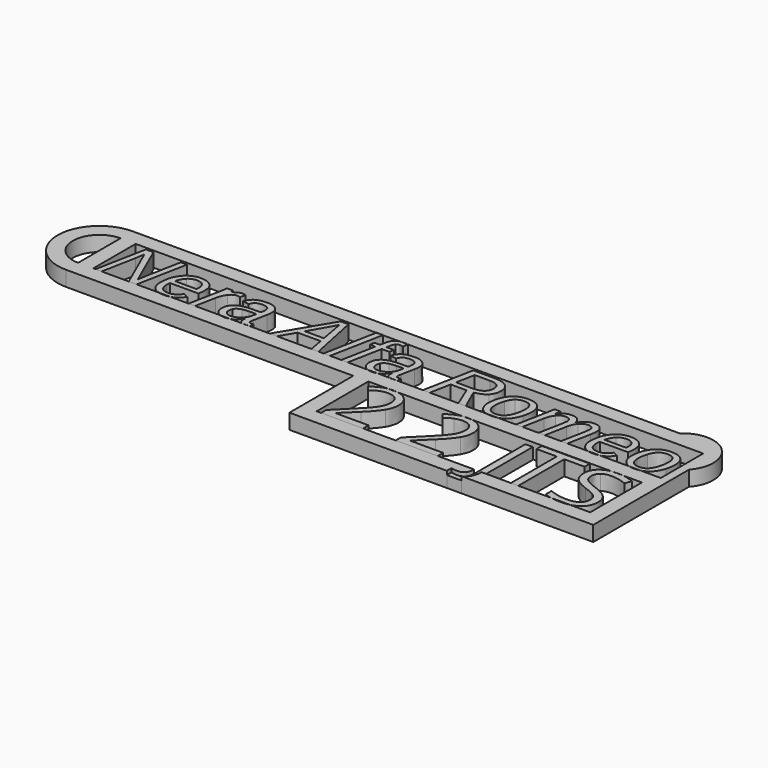
from build123d import *

# Parameters (mm, degrees)
F1_DEPTH = 2
F2_DEPTH = 2
F3_DEPTH = 0.5


with BuildPart() as f1:
    # F0 (on Top) → F1 (new body)
    with BuildSketch(Plane.XY):
        with BuildLine():
            Line((-9.0088317637, 8.9224354902), (-10.3058150991, 2.2276903254))
            Line((-10.3058150991, 2.2276903254), (-9.4984315691, 2.2276903254))
            Line((-9.4984315691, 2.2276903254), (-8.637830669, 6.7085928919))
            add(Edge.make_bspline(
                [(-8.438645655, 7.9766867978), (-8.543559899, 7.1647417789), (-8.637830669, 6.7085928919)],
                knots=[0, 0, 0, 1, 1, 1], degree=2))
            Line((-8.438645655, 7.9766867978), (-5.9161423099, 2.2276903254))
            Line((-5.9161423099, 2.2276903254), (-4.8700408624, 2.2276903254))
            Line((-4.8700408624, 2.2276903254), (-3.573057527, 8.9224354902))
            Line((-3.573057527, 8.9224354902), (-4.3895640347, 8.9224354902))
            Line((-4.3895640347, 8.9224354902), (-5.2501649349, 4.4993117826))
            add(Edge.make_bspline(
                [(-5.4645549118, 3.1491110771), (-5.339874216, 4.0477243845), (-5.2501649349, 4.4993117826)],
                knots=[0, 0, 0, 1, 1, 1], degree=2))
            Line((-5.4645549118, 3.1491110771), (-8.0007427235, 8.9224354902))
            Line((-8.0007427235, 8.9224354902), (-9.0088317637, 8.9224354902))
        make_face()
        with BuildLine():
            add(Edge.make_bspline(
                [(-1.9696861122, 2.2276903254), (-2.4147037445, 2.3571969005), (-2.7192988602, 2.6617920161)],
                knots=[0.4251761387, 0.4251761387, 0.4251761387, 1, 1, 1], degree=2))
            Line((-1.9696861122, 2.2276903254), (-0.4300085657, 2.2276903254))
            add(Edge.make_bspline(
                [(0.0601683579, 2.4177523616), (-0.1648991002, 2.2973748876), (-0.4300085657, 2.2276903254)],
                knots=[0, 0, 0, 0.4211162613, 0.4211162613, 0.4211162613], degree=2))
            add(Edge.make_bspline(
                [(0.941295958, 3.3254886467), (0.5946228038, 2.7036056641), (0.0601683579, 2.4177523616)],
                knots=[0, 0, 0, 1, 1, 1], degree=2))
            Line((0.941295958, 3.3254886467), (0.285962057, 3.6250264159))
            add(Edge.make_bspline(
                [(-0.2994290147, 3.001622937), (0.076133569, 3.2296973805), (0.285962057, 3.6250264159)],
                knots=[0, 0, 0, 1, 1, 1], degree=2))
            add(Edge.make_bspline(
                [(-1.1357019742, 2.7735484935), (-0.6749915983, 2.7735484935), (-0.2994290147, 3.001622937)],
                knots=[0, 0, 0, 1, 1, 1], degree=2))
            add(Edge.make_bspline(
                [(-2.0875326517, 3.1110986698), (-1.7712694234, 2.7735484935), (-1.1357019742, 2.7735484935)],
                knots=[0, 0, 0, 1, 1, 1], degree=2))
            add(Edge.make_bspline(
                [(-2.40379588, 4.0811753028), (-2.40379588, 3.4486488462), (-2.0875326517, 3.1110986698)],
                knots=[0, 0, 0, 1, 1, 1], degree=2))
            add(Edge.make_bspline(
                [(-2.3612219839, 4.6179104932), (-2.3901114134, 4.4521763976), (-2.40379588, 4.0811753028)],
                knots=[0, 0, 0, 1, 1, 1], degree=2))
            Line((-2.3612219839, 4.6179104932), (1.3594324377, 4.6179104932))
            add(Edge.make_bspline(
                [(1.4734696595, 5.5925486151), (1.4734696595, 5.0923053357), (1.3594324377, 4.6179104932)],
                knots=[0, 0, 0, 1, 1, 1], degree=2))
            add(Edge.make_bspline(
                [(0.9314127321, 6.9746797427), (1.4734696595, 6.4850799373), (1.4734696595, 5.5925486151)],
                knots=[0, 0, 0, 1, 1, 1], degree=2))
            add(Edge.make_bspline(
                [(-0.5837618209, 7.4642795481), (0.3893558047, 7.4642795481), (0.9314127321, 6.9746797427)],
                knots=[0, 0, 0, 1, 1, 1], degree=2))
            add(Edge.make_bspline(
                [(-1.9620917078, 7.0438623239), (-1.3485714548, 7.4642795481), (-0.5837618209, 7.4642795481)],
                knots=[0, 0, 0, 1, 1, 1], degree=2))
            add(Edge.make_bspline(
                [(-2.912401889, 5.8654776992), (-2.5756119608, 6.6234450997), (-1.9620917078, 7.0438623239)],
                knots=[0, 0, 0, 1, 1, 1], degree=2))
            add(Edge.make_bspline(
                [(-3.2491918173, 4.1526386285), (-3.2491918173, 5.1075102986), (-2.912401889, 5.8654776992)],
                knots=[0, 0, 0, 1, 1, 1], degree=2))
            add(Edge.make_bspline(
                [(-2.7192988602, 2.6617920161), (-3.2491918173, 3.1916849732), (-3.2491918173, 4.1526386285)],
                knots=[0, 0, 0, 1, 1, 1], degree=2))
        make_face()
        with BuildLine():
            Line((0.6235122334, 5.6153560594), (0.6037457816, 5.2732443942))
            Line((0.6037457816, 5.2732443942), (-2.2471847621, 5.2732443942))
            add(Edge.make_bspline(
                [(-1.6359452536, 6.425780582), (-2.0708071925, 6.0198080726), (-2.2471847621, 5.2732443942)],
                knots=[0, 0, 0, 1, 1, 1], degree=2))
            add(Edge.make_bspline(
                [(-0.5655158654, 6.8317530914), (-1.2010833146, 6.8317530914), (-1.6359452536, 6.425780582)],
                knots=[0, 0, 0, 1, 1, 1], degree=2))
            add(Edge.make_bspline(
                [(0.3163719828, 6.5185308557), (0.0092317322, 6.8317530914), (-0.5655158654, 6.8317530914)],
                knots=[0, 0, 0, 1, 1, 1], degree=2))
            add(Edge.make_bspline(
                [(0.6235122334, 5.6153560594), (0.6235122334, 6.20530862), (0.3163719828, 6.5185308557)],
                knots=[0, 0, 0, 1, 1, 1], degree=2))
        make_face(mode=Mode.SUBTRACT)
        with BuildLine():
            Line((2.7658915059, 6.1718577016), (1.9949998869, 2.2276903254))
            Line((1.9949998869, 2.2276903254), (2.8510392982, 2.2276903254))
            Line((2.8510392982, 2.2276903254), (3.3740900219, 4.9083252846))
            add(Edge.make_bspline(
                [(3.9169071975, 6.2235545754), (3.5154961769, 5.7005038517), (3.3740900219, 4.9083252846)],
                knots=[0, 0, 0, 1, 1, 1], degree=2))
            add(Edge.make_bspline(
                [(4.8185614974, 6.7466052992), (4.318318218, 6.7466052992), (3.9169071975, 6.2235545754)],
                knots=[0, 0, 0, 1, 1, 1], degree=2))
            add(Edge.make_bspline(
                [(5.2458209549, 6.6842649513), (5.0359924669, 6.7466052992), (4.8185614974, 6.7466052992)],
                knots=[0, 0, 0, 1, 1, 1], degree=2))
            Line((5.2458209549, 6.6842649513), (5.4024320728, 7.3973777113))
            add(Edge.make_bspline(
                [(4.9508446747, 7.4642795481), (5.1697961404, 7.4642795481), (5.4024320728, 7.3973777113)],
                knots=[0, 0, 0, 1, 1, 1], degree=2))
            add(Edge.make_bspline(
                [(4.2483753887, 7.2073156751), (4.5524746467, 7.4642795481), (4.9508446747, 7.4642795481)],
                knots=[0, 0, 0, 1, 1, 1], degree=2))
            add(Edge.make_bspline(
                [(4.1290557119, 7.0925359614), (4.1889189826, 7.1570750119), (4.2483753887, 7.2073156751)],
                knots=[0.8044835543, 0.8044835543, 0.8044835543, 1, 1, 1], degree=2))
            add(Edge.make_bspline(
                [(3.6295333987, 6.3193458417), (3.8827387504, 6.8269797595), (4.1290557119, 7.0925359614)],
                knots=[0, 0, 0, 0.8044835543, 0.8044835543, 0.8044835543], degree=2))
            Line((3.6295333987, 6.3193458417), (3.6112874432, 6.3193458417))
            Line((3.6112874432, 6.3193458417), (3.7334290708, 7.0925359614))
            Line((3.7334290708, 7.0925359614), (3.7770215388, 7.3684882818))
            Line((3.7770215388, 7.3684882818), (2.9696380088, 7.3684882818))
            Line((2.9696380088, 7.3684882818), (2.8844902166, 6.8271916026))
            Line((2.8844902166, 6.8271916026), (2.7658915059, 6.1718577016))
        make_face()
        with BuildLine():
            Line((9.0913622365, 2.2276903254), (9.9547242293, 2.2276903254))
            add(Edge.make_bspline(
                [(10.0870811422, 2.2565797549), (10.0204903416, 2.2404169392), (9.9547242293, 2.2276903254)],
                knots=[0, 0, 0, 0.2125992126, 0.2125992126, 0.2125992126], degree=2))
            Line((10.0870811422, 2.2565797549), (10.153982979, 2.7887534564))
            add(Edge.make_bspline(
                [(9.8681296765, 2.755302538), (9.9973718611, 2.755302538), (10.153982979, 2.7887534564)],
                knots=[0, 0, 0, 1, 1, 1], degree=2))
            add(Edge.make_bspline(
                [(9.4834441151, 3.1019756921), (9.4834441151, 2.755302538), (9.8681296765, 2.755302538)],
                knots=[0, 0, 0, 1, 1, 1], degree=2))
            add(Edge.make_bspline(
                [(9.535140989, 3.5201121718), (9.4834441151, 3.2920377283), (9.4834441151, 3.1019756921)],
                knots=[0, 0, 0, 1, 1, 1], degree=2))
            Line((9.535140989, 3.5201121718), (9.8878961283, 5.3158182903))
            add(Edge.make_bspline(
                [(9.9776054094, 6.0623819687), (9.9776054094, 5.7582827107), (9.8878961283, 5.3158182903)],
                knots=[0, 0, 0, 1, 1, 1], degree=2))
            add(Edge.make_bspline(
                [(9.5047310632, 7.0841554756), (9.9776054094, 6.7040314031), (9.9776054094, 6.0623819687)],
                knots=[0, 0, 0, 1, 1, 1], degree=2))
            add(Edge.make_bspline(
                [(8.2199116981, 7.4642795481), (9.031856717, 7.4642795481), (9.5047310632, 7.0841554756)],
                knots=[0, 0, 0, 1, 1, 1], degree=2))
            add(Edge.make_bspline(
                [(6.7959669226, 7.1480163198), (7.3258598796, 7.4642795481), (8.2199116981, 7.4642795481)],
                knots=[0, 0, 0, 1, 1, 1], degree=2))
            add(Edge.make_bspline(
                [(6.0532044849, 6.1338452943), (6.2660739655, 6.8317530914), (6.7959669226, 7.1480163198)],
                knots=[0, 0, 0, 1, 1, 1], degree=2))
            Line((6.0532044849, 6.1338452943), (6.8986004221, 5.9954801319))
            add(Edge.make_bspline(
                [(7.3167369019, 6.6112811294), (7.0263221105, 6.4090551228), (6.8986004221, 5.9954801319)],
                knots=[0, 0, 0, 1, 1, 1], degree=2))
            add(Edge.make_bspline(
                [(8.1727763131, 6.813507136), (7.6071516933, 6.813507136), (7.3167369019, 6.6112811294)],
                knots=[0, 0, 0, 1, 1, 1], degree=2))
            add(Edge.make_bspline(
                [(8.8706841103, 6.6067196405), (8.6182817261, 6.813507136), (8.1727763131, 6.813507136)],
                knots=[0, 0, 0, 1, 1, 1], degree=2))
            add(Edge.make_bspline(
                [(9.1230864944, 5.9665907024), (9.1230864944, 6.3999321451), (8.8706841103, 6.6067196405)],
                knots=[0, 0, 0, 1, 1, 1], degree=2))
            add(Edge.make_bspline(
                [(9.031856717, 5.3644741716), (9.1230864944, 5.8297460363), (9.1230864944, 5.9665907024)],
                knots=[0, 0, 0, 1, 1, 1], degree=2))
            Line((9.031856717, 5.3644741716), (7.9294969067, 5.3492692087))
            add(Edge.make_bspline(
                [(5.922441804, 4.8794358551), (6.551927268, 5.3310232532), (7.9294969067, 5.3492692087)],
                knots=[0, 0, 0, 1, 1, 1], degree=2))
            add(Edge.make_bspline(
                [(5.2929563399, 3.5490016014), (5.2929563399, 4.427848457), (5.922441804, 4.8794358551)],
                knots=[0, 0, 0, 1, 1, 1], degree=2))
            add(Edge.make_bspline(
                [(5.7088120752, 2.5317895833), (5.2929563399, 2.9316801076), (5.2929563399, 3.5490016014)],
                knots=[0, 0, 0, 1, 1, 1], degree=2))
            add(Edge.make_bspline(
                [(6.1982625562, 2.2276903254), (5.9211346878, 2.327618296), (5.7088120752, 2.5317895833)],
                knots=[0.4894320446, 0.4894320446, 0.4894320446, 1, 1, 1], degree=2))
            Line((6.1982625562, 2.2276903254), (7.4753742359, 2.2276903254))
            add(Edge.make_bspline(
                [(7.8108981961, 2.3721374729), (7.6551145583, 2.2835985708), (7.4753742359, 2.2276903254)],
                knots=[0, 0, 0, 0.3685459817, 0.3685459817, 0.3685459817], degree=2))
            add(Edge.make_bspline(
                [(8.6289252001, 3.211451425), (8.2335961647, 2.6123758867), (7.8108981961, 2.3721374729)],
                knots=[0, 0, 0, 1, 1, 1], degree=2))
            Line((8.6289252001, 3.211451425), (8.6562941334, 3.211451425))
            Line((8.6562941334, 3.211451425), (8.633486689, 2.907352167))
            add(Edge.make_bspline(
                [(8.8349524474, 2.3630144952), (8.633486689, 2.54547405), (8.633486689, 2.907352167)],
                knots=[0, 0, 0, 1, 1, 1], degree=2))
            add(Edge.make_bspline(
                [(9.0913622365, 2.2276903254), (8.9340202076, 2.2732927501), (8.8349524474, 2.3630144952)],
                knots=[0.5082650227, 0.5082650227, 0.5082650227, 1, 1, 1], degree=2))
        make_face()
        with BuildLine():
            Line((7.9720708029, 4.7562756556), (8.9178194952, 4.7745216111))
            Line((8.9178194952, 4.7745216111), (8.7900978069, 4.1800075617))
            add(Edge.make_bspline(
                [(8.4715538341, 3.4965444793), (8.7140729924, 3.8150884521), (8.7900978069, 4.1800075617)],
                knots=[0, 0, 0, 1, 1, 1], degree=2))
            add(Edge.make_bspline(
                [(7.8587938293, 2.981096237), (8.2290346759, 3.1780005066), (8.4715538341, 3.4965444793)],
                knots=[0, 0, 0, 1, 1, 1], degree=2))
            add(Edge.make_bspline(
                [(7.0263221105, 2.7841919675), (7.4885529827, 2.7841919675), (7.8587938293, 2.981096237)],
                knots=[0, 0, 0, 1, 1, 1], degree=2))
            add(Edge.make_bspline(
                [(6.431047813, 3.006944674), (6.6614030009, 2.7841919675), (7.0263221105, 2.7841919675)],
                knots=[0, 0, 0, 1, 1, 1], degree=2))
            add(Edge.make_bspline(
                [(6.200692625, 3.5870140086), (6.200692625, 3.2296973805), (6.431047813, 3.006944674)],
                knots=[0, 0, 0, 1, 1, 1], degree=2))
            add(Edge.make_bspline(
                [(6.3025658765, 4.0880175362), (6.200692625, 3.8819902889), (6.200692625, 3.5870140086)],
                knots=[0, 0, 0, 1, 1, 1], degree=2))
            add(Edge.make_bspline(
                [(6.5823371938, 4.4301292014), (6.4044391279, 4.2940447834), (6.3025658765, 4.0880175362)],
                knots=[0, 0, 0, 1, 1, 1], degree=2))
            add(Edge.make_bspline(
                [(7.0833407214, 4.653642156), (6.7602352597, 4.5662136194), (6.5823371938, 4.4301292014)],
                knots=[0, 0, 0, 1, 1, 1], degree=2))
            add(Edge.make_bspline(
                [(7.9720708029, 4.7562756556), (7.406446183, 4.7410706927), (7.0833407214, 4.653642156)],
                knots=[0, 0, 0, 1, 1, 1], degree=2))
        make_face(mode=Mode.SUBTRACT)
        Polygon((18.2308592714, 2.2276903254), (19.156841512, 2.2276903254), (17.7701488956, 8.9224354902), (16.7377319147, 8.9224354902), (12.7084167462, 2.2276903254), (13.6967393347, 2.2276903254), (14.8371115522, 4.1860895469), (17.8735426433, 4.1860895469), align=None)
        with BuildLine():
            add(Edge.make_bspline(
                [(17.1330609501, 8.2382121597), (17.0707206022, 8.1150519602), (16.9566833804, 7.9105452092)],
                knots=[0, 0, 0, 1, 1, 1], degree=2))
            Line((17.1330609501, 8.2382121597), (17.2562211495, 7.5205379108))
            Line((17.2562211495, 7.5205379108), (17.741259466, 4.8931203217))
            Line((17.741259466, 4.8931203217), (15.2370020764, 4.8931203217))
            add(Edge.make_bspline(
                [(16.9566833804, 7.9105452092), (16.8426461587, 7.7060384582), (15.2370020764, 4.8931203217)],
                knots=[0, 0, 0, 1, 1, 1], degree=2))
        make_face(mode=Mode.SUBTRACT)
        Polygon((22.05210839, 9.2341372296), (21.1960984838, 9.2341372296), (19.8365033537, 2.2276903254), (20.687981276, 2.2276903254), align=None)
        with BuildLine():
            Line((25.3320137021, 9.2341372296), (24.3199696419, 9.2341372296))
            add(Edge.make_bspline(
                [(24.0421960918, 9.1436677004), (24.1663926885, 9.2009645839), (24.3199696419, 9.2341372296)],
                knots=[0, 0, 0, 0.4210392667, 0.4210392667, 0.4210392667], degree=2))
            add(Edge.make_bspline(
                [(23.5693217456, 8.7445374242), (23.7472198115, 9.0075832824), (24.0421960918, 9.1436677004)],
                knots=[0, 0, 0, 1, 1, 1], degree=2))
            add(Edge.make_bspline(
                [(23.2819479468, 7.9493178646), (23.3914236796, 8.4814915661), (23.5693217456, 8.7445374242)],
                knots=[0, 0, 0, 1, 1, 1], degree=2))
            Line((23.2819479468, 7.9493178646), (23.1724722139, 7.3684882818))
            Line((23.1724722139, 7.3684882818), (22.4502364761, 7.3684882818))
            Line((22.4502364761, 7.3684882818), (22.3270762767, 6.7466052992))
            Line((22.3270762767, 6.7466052992), (23.0493120144, 6.7466052992))
            Line((23.0493120144, 6.7466052992), (22.1704651588, 2.2276903254))
            Line((22.1704651588, 2.2276903254), (23.0249840738, 2.2276903254))
            Line((23.0249840738, 2.2276903254), (23.9038309294, 6.7466052992))
            Line((23.9038309294, 6.7466052992), (24.9073584808, 6.7466052992))
            Line((24.9073584808, 6.7466052992), (25.0305186803, 7.3684882818))
            Line((25.0305186803, 7.3684882818), (24.0285116252, 7.3684882818))
            Line((24.0285116252, 7.3684882818), (24.1182209063, 7.8291986577))
            add(Edge.make_bspline(
                [(24.3721437867, 8.454882881), (24.2124916762, 8.3005525076), (24.1182209063, 7.8291986577)],
                knots=[0, 0, 0, 1, 1, 1], degree=2))
            add(Edge.make_bspline(
                [(24.8313336663, 8.6092132544), (24.5317958971, 8.6092132544), (24.3721437867, 8.454882881)],
                knots=[0, 0, 0, 1, 1, 1], degree=2))
            Line((24.8313336663, 8.6092132544), (25.0487646357, 8.6000902767))
            Line((25.0487646357, 8.6000902767), (25.2631546126, 8.5712008472))
            Line((25.2631546126, 8.5712008472), (25.3863148121, 9.2219732593))
            add(Edge.make_bspline(
                [(25.3320137021, 9.2341372296), (25.3598728303, 9.2284142549), (25.3863148121, 9.2219732593)],
                knots=[0.8885233166, 0.8885233166, 0.8885233166, 1, 1, 1], degree=2))
        make_face()
        with BuildLine():
            add(Edge.make_bspline(
                [(25.6697380458, 2.2276903254), (25.3926101774, 2.327618296), (25.1802875648, 2.5317895833)],
                knots=[0.4894320446, 0.4894320446, 0.4894320446, 1, 1, 1], degree=2))
            Line((25.6697380458, 2.2276903254), (26.9468497255, 2.2276903254))
            add(Edge.make_bspline(
                [(27.2823736857, 2.3721374729), (27.1265900479, 2.2835985708), (26.9468497255, 2.2276903254)],
                knots=[0, 0, 0, 0.3685459817, 0.3685459817, 0.3685459817], degree=2))
            add(Edge.make_bspline(
                [(28.1004006897, 3.211451425), (27.7050716543, 2.6123758867), (27.2823736857, 2.3721374729)],
                knots=[0, 0, 0, 1, 1, 1], degree=2))
            Line((28.1004006897, 3.211451425), (28.127769623, 3.211451425))
            Line((28.127769623, 3.211451425), (28.1049621786, 2.907352167))
            add(Edge.make_bspline(
                [(28.306427937, 2.3630144952), (28.1049621786, 2.54547405), (28.1049621786, 2.907352167)],
                knots=[0, 0, 0, 1, 1, 1], degree=2))
            add(Edge.make_bspline(
                [(28.5628377261, 2.2276903254), (28.4054956972, 2.2732927501), (28.306427937, 2.3630144952)],
                knots=[0.5082650227, 0.5082650227, 0.5082650227, 1, 1, 1], degree=2))
            Line((28.5628377261, 2.2276903254), (29.4261997189, 2.2276903254))
            add(Edge.make_bspline(
                [(29.5585566318, 2.2565797549), (29.4919658312, 2.2404169392), (29.4261997189, 2.2276903254)],
                knots=[0, 0, 0, 0.2125992126, 0.2125992126, 0.2125992126], degree=2))
            Line((29.5585566318, 2.2565797549), (29.6254584686, 2.7887534564))
            add(Edge.make_bspline(
                [(29.3396051661, 2.755302538), (29.4688473507, 2.755302538), (29.6254584686, 2.7887534564)],
                knots=[0, 0, 0, 1, 1, 1], degree=2))
            add(Edge.make_bspline(
                [(28.9549196047, 3.1019756921), (28.9549196047, 2.755302538), (29.3396051661, 2.755302538)],
                knots=[0, 0, 0, 1, 1, 1], degree=2))
            add(Edge.make_bspline(
                [(29.0066164786, 3.5201121718), (28.9549196047, 3.2920377283), (28.9549196047, 3.1019756921)],
                knots=[0, 0, 0, 1, 1, 1], degree=2))
            Line((29.0066164786, 3.5201121718), (29.3593716179, 5.3158182903))
            add(Edge.make_bspline(
                [(29.449080899, 6.0623819687), (29.449080899, 5.7582827107), (29.3593716179, 5.3158182903)],
                knots=[0, 0, 0, 1, 1, 1], degree=2))
            add(Edge.make_bspline(
                [(28.9762065528, 7.0841554756), (29.449080899, 6.7040314031), (29.449080899, 6.0623819687)],
                knots=[0, 0, 0, 1, 1, 1], degree=2))
            add(Edge.make_bspline(
                [(27.6913871877, 7.4642795481), (28.5033322066, 7.4642795481), (28.9762065528, 7.0841554756)],
                knots=[0, 0, 0, 1, 1, 1], degree=2))
            add(Edge.make_bspline(
                [(26.2674424122, 7.1480163198), (26.7973353692, 7.4642795481), (27.6913871877, 7.4642795481)],
                knots=[0, 0, 0, 1, 1, 1], degree=2))
            add(Edge.make_bspline(
                [(25.5246799745, 6.1338452943), (25.7375494551, 6.8317530914), (26.2674424122, 7.1480163198)],
                knots=[0, 0, 0, 1, 1, 1], degree=2))
            Line((25.5246799745, 6.1338452943), (26.3700759117, 5.9954801319))
            add(Edge.make_bspline(
                [(26.7882123915, 6.6112811294), (26.4977976001, 6.4090551228), (26.3700759117, 5.9954801319)],
                knots=[0, 0, 0, 1, 1, 1], degree=2))
            add(Edge.make_bspline(
                [(27.6442518027, 6.813507136), (27.0786271829, 6.813507136), (26.7882123915, 6.6112811294)],
                knots=[0, 0, 0, 1, 1, 1], degree=2))
            add(Edge.make_bspline(
                [(28.3421595999, 6.6067196405), (28.0897572157, 6.813507136), (27.6442518027, 6.813507136)],
                knots=[0, 0, 0, 1, 1, 1], degree=2))
            add(Edge.make_bspline(
                [(28.594561984, 5.9665907024), (28.594561984, 6.3999321451), (28.3421595999, 6.6067196405)],
                knots=[0, 0, 0, 1, 1, 1], degree=2))
            add(Edge.make_bspline(
                [(28.5033322066, 5.3644741716), (28.594561984, 5.8297460363), (28.594561984, 5.9665907024)],
                knots=[0, 0, 0, 1, 1, 1], degree=2))
            Line((28.5033322066, 5.3644741716), (27.4009723963, 5.3492692087))
            add(Edge.make_bspline(
                [(25.3939172936, 4.8794358551), (26.0234027576, 5.3310232532), (27.4009723963, 5.3492692087)],
                knots=[0, 0, 0, 1, 1, 1], degree=2))
            add(Edge.make_bspline(
                [(24.7644318295, 3.5490016014), (24.7644318295, 4.427848457), (25.3939172936, 4.8794358551)],
                knots=[0, 0, 0, 1, 1, 1], degree=2))
            add(Edge.make_bspline(
                [(25.1802875648, 2.5317895833), (24.7644318295, 2.9316801076), (24.7644318295, 3.5490016014)],
                knots=[0, 0, 0, 1, 1, 1], degree=2))
        make_face()
        with BuildLine():
            Line((27.4435462925, 4.7562756556), (28.3892949848, 4.7745216111))
            Line((28.3892949848, 4.7745216111), (28.2615732965, 4.1800075617))
            add(Edge.make_bspline(
                [(27.9430293237, 3.4965444793), (28.185548482, 3.8150884521), (28.2615732965, 4.1800075617)],
                knots=[0, 0, 0, 1, 1, 1], degree=2))
            add(Edge.make_bspline(
                [(27.3302693189, 2.981096237), (27.7005101655, 3.1780005066), (27.9430293237, 3.4965444793)],
                knots=[0, 0, 0, 1, 1, 1], degree=2))
            add(Edge.make_bspline(
                [(26.4977976001, 2.7841919675), (26.9600284723, 2.7841919675), (27.3302693189, 2.981096237)],
                knots=[0, 0, 0, 1, 1, 1], degree=2))
            add(Edge.make_bspline(
                [(25.9025233026, 3.006944674), (26.1328784905, 2.7841919675), (26.4977976001, 2.7841919675)],
                knots=[0, 0, 0, 1, 1, 1], degree=2))
            add(Edge.make_bspline(
                [(25.6721681146, 3.5870140086), (25.6721681146, 3.2296973805), (25.9025233026, 3.006944674)],
                knots=[0, 0, 0, 1, 1, 1], degree=2))
            add(Edge.make_bspline(
                [(25.7740413661, 4.0880175362), (25.6721681146, 3.8819902889), (25.6721681146, 3.5870140086)],
                knots=[0, 0, 0, 1, 1, 1], degree=2))
            add(Edge.make_bspline(
                [(26.0538126834, 4.4301292014), (25.8759146175, 4.2940447834), (25.7740413661, 4.0880175362)],
                knots=[0, 0, 0, 1, 1, 1], degree=2))
            add(Edge.make_bspline(
                [(26.554816211, 4.653642156), (26.2317107493, 4.5662136194), (26.0538126834, 4.4301292014)],
                knots=[0, 0, 0, 1, 1, 1], degree=2))
            add(Edge.make_bspline(
                [(27.4435462925, 4.7562756556), (26.8779216726, 4.7410706927), (26.554816211, 4.653642156)],
                knots=[0, 0, 0, 1, 1, 1], degree=2))
        make_face(mode=Mode.SUBTRACT)
        with BuildLine():
            Line((34.2568901679, 8.9224354902), (32.9599068325, 2.2276903254))
            Line((32.9599068325, 2.2276903254), (33.8676431177, 2.2276903254))
            Line((33.8676431177, 2.2276903254), (34.404378308, 5.0071575435))
            Line((34.404378308, 5.0071575435), (36.4996221956, 5.0071575435))
            Line((36.4996221956, 5.0071575435), (37.6536788797, 2.2276903254))
            Line((37.6536788797, 2.2276903254), (38.6328784905, 2.2276903254))
            Line((38.6328784905, 2.2276903254), (37.3602230958, 5.0877438468))
            add(Edge.make_bspline(
                [(38.8753976488, 5.7483994848), (38.3622301509, 5.2261090092), (37.3602230958, 5.0877438468)],
                knots=[0, 0, 0, 1, 1, 1], degree=2))
            add(Edge.make_bspline(
                [(39.3885651466, 7.1647417789), (39.3885651466, 6.2706899604), (38.8753976488, 5.7483994848)],
                knots=[0, 0, 0, 1, 1, 1], degree=2))
            add(Edge.make_bspline(
                [(38.7849281195, 8.4381574218), (39.3885651466, 7.9538793535), (39.3885651466, 7.1647417789)],
                knots=[0, 0, 0, 1, 1, 1], degree=2))
            add(Edge.make_bspline(
                [(37.1655995707, 8.9224354902), (38.1812910924, 8.9224354902), (38.7849281195, 8.4381574218)],
                knots=[0, 0, 0, 1, 1, 1], degree=2))
            Line((37.1655995707, 8.9224354902), (34.2568901679, 8.9224354902))
        make_face()
        with BuildLine():
            add(Edge.make_bspline(
                [(36.732258128, 5.7248317923), (37.5928590281, 5.7248317923), (38.0300017115, 6.0836689168)],
                knots=[0, 0, 0, 1, 1, 1], degree=2))
            Line((36.732258128, 5.7248317923), (34.5473049593, 5.7248317923))
            Line((34.5473049593, 5.7248317923), (35.0262612906, 8.1956382636))
            Line((35.0262612906, 8.1956382636), (37.0561238378, 8.1956382636))
            add(Edge.make_bspline(
                [(38.1128687593, 7.9105452092), (37.7585931238, 8.1956382636), (37.0561238378, 8.1956382636)],
                knots=[0, 0, 0, 1, 1, 1], degree=2))
            add(Edge.make_bspline(
                [(38.4671443949, 7.0932784533), (38.4671443949, 7.6254521548), (38.1128687593, 7.9105452092)],
                knots=[0, 0, 0, 1, 1, 1], degree=2))
            add(Edge.make_bspline(
                [(38.0300017115, 6.0836689168), (38.4671443949, 6.4425060412), (38.4671443949, 7.0932784533)],
                knots=[0, 0, 0, 1, 1, 1], degree=2))
        make_face(mode=Mode.SUBTRACT)
        with BuildLine():
            add(Edge.make_bspline(
                [(41.3178756053, 2.2276903254), (40.866024234, 2.3637286253), (40.5479435677, 2.6929621901)],
                knots=[0.4131969353, 0.4131969353, 0.4131969353, 1, 1, 1], degree=2))
            Line((41.3178756053, 2.2276903254), (42.8067506557, 2.2276903254))
            add(Edge.make_bspline(
                [(43.1905661197, 2.3630144952), (43.0077739616, 2.2806903232), (42.8067506557, 2.2276903254)],
                knots=[0, 0, 0, 0.3562036935, 0.3562036935, 0.3562036935], degree=2))
            add(Edge.make_bspline(
                [(44.057249005, 3.0571210515), (43.7037336176, 2.5941299312), (43.1905661197, 2.3630144952)],
                knots=[0, 0, 0, 1, 1, 1], degree=2))
            add(Edge.make_bspline(
                [(44.6008264287, 4.1876100431), (44.4107643925, 3.5201121718), (44.057249005, 3.0571210515)],
                knots=[0, 0, 0, 1, 1, 1], degree=2))
            add(Edge.make_bspline(
                [(44.790888465, 5.4724294082), (44.790888465, 4.8551079145), (44.6008264287, 4.1876100431)],
                knots=[0, 0, 0, 1, 1, 1], degree=2))
            add(Edge.make_bspline(
                [(44.2640365005, 6.9389480799), (44.790888465, 6.4181781006), (44.790888465, 5.4724294082)],
                knots=[0, 0, 0, 1, 1, 1], degree=2))
            add(Edge.make_bspline(
                [(42.7382184735, 7.4597180592), (43.737184536, 7.4597180592), (44.2640365005, 6.9389480799)],
                knots=[0, 0, 0, 1, 1, 1], degree=2))
            add(Edge.make_bspline(
                [(41.2793022832, 7.0742722497), (41.8684945956, 7.4597180592), (42.7382184735, 7.4597180592)],
                knots=[0, 0, 0, 1, 1, 1], degree=2))
            add(Edge.make_bspline(
                [(40.3578815315, 5.9384615211), (40.6901099709, 6.6888264402), (41.2793022832, 7.0742722497)],
                knots=[0, 0, 0, 1, 1, 1], degree=2))
            add(Edge.make_bspline(
                [(40.0058866404, 4.2180199689), (40.0256530921, 5.188096602), (40.3578815315, 5.9384615211)],
                knots=[0, 0, 0, 1, 1, 1], degree=2))
            add(Edge.make_bspline(
                [(40.5479435677, 2.6929621901), (40.0058866404, 3.2540253211), (40.0058866404, 4.2180199689)],
                knots=[0, 0, 0, 1, 1, 1], degree=2))
        make_face()
        with BuildLine():
            add(Edge.make_bspline(
                [(43.9074801205, 5.4724294082), (43.9074801205, 6.8317530914), (42.7290954957, 6.8317530914)],
                knots=[0, 0, 0, 1, 1, 1], degree=2))
            add(Edge.make_bspline(
                [(43.7432665212, 4.3328174388), (43.8831521798, 4.8748743662), (43.9074801205, 5.4724294082)],
                knots=[0, 0, 0, 1, 1, 1], degree=2))
            add(Edge.make_bspline(
                [(43.3798679078, 3.4418066129), (43.6033808625, 3.7907605115), (43.7432665212, 4.3328174388)],
                knots=[0, 0, 0, 1, 1, 1], degree=2))
            add(Edge.make_bspline(
                [(42.8598581767, 2.928639115), (43.1563549532, 3.0928527144), (43.3798679078, 3.4418066129)],
                knots=[0, 0, 0, 1, 1, 1], degree=2))
            add(Edge.make_bspline(
                [(42.0737615947, 2.7644255157), (42.5633614001, 2.7644255157), (42.8598581767, 2.928639115)],
                knots=[0, 0, 0, 1, 1, 1], degree=2))
            add(Edge.make_bspline(
                [(41.1903532503, 3.133145866), (41.4944525083, 2.7644255157), (42.0737615947, 2.7644255157)],
                knots=[0, 0, 0, 1, 1, 1], degree=2))
            add(Edge.make_bspline(
                [(40.8862539923, 4.2043355023), (40.8862539923, 3.5018662164), (41.1903532503, 3.133145866)],
                knots=[0, 0, 0, 1, 1, 1], degree=2))
            add(Edge.make_bspline(
                [(41.099883721, 5.5020790858), (40.8862539923, 4.8323004701), (40.8862539923, 4.2043355023)],
                knots=[0, 0, 0, 1, 1, 1], degree=2))
            add(Edge.make_bspline(
                [(41.7004797556, 6.5018053965), (41.3135134497, 6.1718577016), (41.099883721, 5.5020790858)],
                knots=[0, 0, 0, 1, 1, 1], degree=2))
            add(Edge.make_bspline(
                [(42.7290954957, 6.8317530914), (42.0874460614, 6.8317530914), (41.7004797556, 6.5018053965)],
                knots=[0, 0, 0, 1, 1, 1], degree=2))
        make_face(mode=Mode.SUBTRACT)
        with BuildLine():
            Line((51.2058623124, 2.2276903254), (52.0512582497, 2.2276903254))
            Line((52.0512582497, 2.2276903254), (52.6548952768, 5.3310232532))
            add(Edge.make_bspline(
                [(52.7537275356, 6.1095173537), (52.7537275356, 5.8054180957), (52.6548952768, 5.3310232532)],
                knots=[0, 0, 0, 1, 1, 1], degree=2))
            add(Edge.make_bspline(
                [(52.4093351259, 7.1122846569), (52.7537275356, 6.7648512547), (52.7537275356, 6.1095173537)],
                knots=[0, 0, 0, 1, 1, 1], degree=2))
            add(Edge.make_bspline(
                [(51.4232932819, 7.4597180592), (52.0649427163, 7.4597180592), (52.4093351259, 7.1122846569)],
                knots=[0, 0, 0, 1, 1, 1], degree=2))
            add(Edge.make_bspline(
                [(50.5467271707, 7.217198901), (50.9291319876, 7.4597180592), (51.4232932819, 7.4597180592)],
                knots=[0, 0, 0, 1, 1, 1], degree=2))
            add(Edge.make_bspline(
                [(49.7705138147, 6.357358249), (50.1643223538, 6.9746797427), (50.5467271707, 7.217198901)],
                knots=[0, 0, 0, 1, 1, 1], degree=2))
            add(Edge.make_bspline(
                [(49.3660618015, 7.1769057493), (49.7036119779, 6.8940934393), (49.7705138147, 6.357358249)],
                knots=[0, 0, 0, 1, 1, 1], degree=2))
            add(Edge.make_bspline(
                [(48.4537640275, 7.4597180592), (49.0285116252, 7.4597180592), (49.3660618015, 7.1769057493)],
                knots=[0, 0, 0, 1, 1, 1], degree=2))
            add(Edge.make_bspline(
                [(47.6205320606, 7.2453280823), (47.9702462073, 7.4597180592), (48.4537640275, 7.4597180592)],
                knots=[0, 0, 0, 1, 1, 1], degree=2))
            add(Edge.make_bspline(
                [(46.9241447598, 6.4896414262), (47.2708179139, 7.0309381054), (47.6205320606, 7.2453280823)],
                knots=[0, 0, 0, 1, 1, 1], degree=2))
            Line((46.9241447598, 6.4896414262), (46.9104602932, 6.4896414262))
            add(Edge.make_bspline(
                [(46.993327341, 7.0005281796), (46.9439112116, 6.6842649513), (46.9104602932, 6.4896414262)],
                knots=[0, 0, 0, 1, 1, 1], degree=2))
            add(Edge.make_bspline(
                [(47.0427434704, 7.3684882818), (47.0427434704, 7.3167914079), (46.993327341, 7.0005281796)],
                knots=[0, 0, 0, 1, 1, 1], degree=2))
            Line((47.0427434704, 7.3684882818), (46.2353599404, 7.3684882818))
            add(Edge.make_bspline(
                [(46.0498593931, 6.2706899604), (46.1456506593, 6.7222773586), (46.2353599404, 7.3684882818)],
                knots=[0, 0, 0, 1, 1, 1], degree=2))
            Line((46.0498593931, 6.2706899604), (45.2607218186, 2.2276903254))
            Line((45.2607218186, 2.2276903254), (46.112199741, 2.2276903254))
            Line((46.112199741, 2.2276903254), (46.6717423757, 5.0983873209))
            add(Edge.make_bspline(
                [(47.2115185586, 6.3284688195), (46.8009845603, 5.8586354658), (46.6717423757, 5.0983873209)],
                knots=[0, 0, 0, 1, 1, 1], degree=2))
            add(Edge.make_bspline(
                [(48.1739927102, 6.7983021731), (47.6220525569, 6.7983021731), (47.2115185586, 6.3284688195)],
                knots=[0, 0, 0, 1, 1, 1], degree=2))
            add(Edge.make_bspline(
                [(48.7631850225, 6.6105208812), (48.5830062122, 6.7983021731), (48.1739927102, 6.7983021731)],
                knots=[0, 0, 0, 1, 1, 1], degree=2))
            add(Edge.make_bspline(
                [(48.9433638329, 6.0669434576), (48.9433638329, 6.4227395894), (48.7631850225, 6.6105208812)],
                knots=[0, 0, 0, 1, 1, 1], degree=2))
            add(Edge.make_bspline(
                [(48.8247651223, 5.2397934758), (48.9433638329, 5.8343075252), (48.9433638329, 6.0669434576)],
                knots=[0, 0, 0, 1, 1, 1], degree=2))
            Line((48.8247651223, 5.2397934758), (48.2363330581, 2.2276903254))
            Line((48.2363330581, 2.2276903254), (49.0817289953, 2.2276903254))
            Line((49.0817289953, 2.2276903254), (49.6427921263, 5.1120717875))
            add(Edge.make_bspline(
                [(50.1840888055, 6.3353110528), (49.7750753035, 5.8723199325), (49.6427921263, 5.1120717875)],
                knots=[0, 0, 0, 1, 1, 1], degree=2))
            add(Edge.make_bspline(
                [(51.1435219645, 6.7983021731), (50.5931023076, 6.7983021731), (50.1840888055, 6.3353110528)],
                knots=[0, 0, 0, 1, 1, 1], degree=2))
            add(Edge.make_bspline(
                [(51.7327142769, 6.6105208812), (51.5525354665, 6.7983021731), (51.1435219645, 6.7983021731)],
                knots=[0, 0, 0, 1, 1, 1], degree=2))
            add(Edge.make_bspline(
                [(51.9128930873, 6.0669434576), (51.9128930873, 6.4227395894), (51.7327142769, 6.6105208812)],
                knots=[0, 0, 0, 1, 1, 1], degree=2))
            add(Edge.make_bspline(
                [(51.7942943766, 5.2397934758), (51.9128930873, 5.8343075252), (51.9128930873, 6.0669434576)],
                knots=[0, 0, 0, 1, 1, 1], degree=2))
            Line((51.7942943766, 5.2397934758), (51.2058623124, 2.2276903254))
        make_face()
        with BuildLine():
            Line((54.8132478375, 2.2276903254), (56.3529253839, 2.2276903254))
            add(Edge.make_bspline(
                [(56.8431023076, 2.4177523616), (56.6180348495, 2.2973748876), (56.3529253839, 2.2276903254)],
                knots=[0, 0, 0, 0.4211162613, 0.4211162613, 0.4211162613], degree=2))
            add(Edge.make_bspline(
                [(57.7242299076, 3.3254886467), (57.3775567535, 2.7036056641), (56.8431023076, 2.4177523616)],
                knots=[0, 0, 0, 1, 1, 1], degree=2))
            Line((57.7242299076, 3.3254886467), (57.0688960066, 3.6250264159))
            add(Edge.make_bspline(
                [(56.483504935, 3.001622937), (56.8590675186, 3.2296973805), (57.0688960066, 3.6250264159)],
                knots=[0, 0, 0, 1, 1, 1], degree=2))
            add(Edge.make_bspline(
                [(55.6472319755, 2.7735484935), (56.1079423513, 2.7735484935), (56.483504935, 3.001622937)],
                knots=[0, 0, 0, 1, 1, 1], degree=2))
            add(Edge.make_bspline(
                [(54.6954012979, 3.1110986698), (55.0116645263, 2.7735484935), (55.6472319755, 2.7735484935)],
                knots=[0, 0, 0, 1, 1, 1], degree=2))
            add(Edge.make_bspline(
                [(54.3791380696, 4.0811753028), (54.3791380696, 3.4486488462), (54.6954012979, 3.1110986698)],
                knots=[0, 0, 0, 1, 1, 1], degree=2))
            add(Edge.make_bspline(
                [(54.4217119657, 4.6179104932), (54.3928225362, 4.4521763976), (54.3791380696, 4.0811753028)],
                knots=[0, 0, 0, 1, 1, 1], degree=2))
            Line((54.4217119657, 4.6179104932), (58.1423663873, 4.6179104932))
            add(Edge.make_bspline(
                [(58.2564036091, 5.5925486151), (58.2564036091, 5.0923053357), (58.1423663873, 4.6179104932)],
                knots=[0, 0, 0, 1, 1, 1], degree=2))
            add(Edge.make_bspline(
                [(57.7143466817, 6.9746797427), (58.2564036091, 6.4850799373), (58.2564036091, 5.5925486151)],
                knots=[0, 0, 0, 1, 1, 1], degree=2))
            add(Edge.make_bspline(
                [(56.1991721287, 7.4642795481), (57.1722897543, 7.4642795481), (57.7143466817, 6.9746797427)],
                knots=[0, 0, 0, 1, 1, 1], degree=2))
            add(Edge.make_bspline(
                [(54.8208422419, 7.0438623239), (55.4343624949, 7.4642795481), (56.1991721287, 7.4642795481)],
                knots=[0, 0, 0, 1, 1, 1], degree=2))
            add(Edge.make_bspline(
                [(53.8705320606, 5.8654776992), (54.2073219889, 6.6234450997), (54.8208422419, 7.0438623239)],
                knots=[0, 0, 0, 1, 1, 1], degree=2))
            add(Edge.make_bspline(
                [(53.5337421324, 4.1526386285), (53.5337421324, 5.1075102986), (53.8705320606, 5.8654776992)],
                knots=[0, 0, 0, 1, 1, 1], degree=2))
            add(Edge.make_bspline(
                [(54.0636350895, 2.6617920161), (53.5337421324, 3.1916849732), (53.5337421324, 4.1526386285)],
                knots=[0, 0, 0, 1, 1, 1], degree=2))
            add(Edge.make_bspline(
                [(54.8132478375, 2.2276903254), (54.3682302051, 2.3571969005), (54.0636350895, 2.6617920161)],
                knots=[0.4251761387, 0.4251761387, 0.4251761387, 1, 1, 1], degree=2))
        make_face()
        with BuildLine():
            Line((57.406446183, 5.6153560594), (57.3866797312, 5.2732443942))
            Line((57.3866797312, 5.2732443942), (54.5357491875, 5.2732443942))
            add(Edge.make_bspline(
                [(55.1469886961, 6.425780582), (54.7121267571, 6.0198080726), (54.5357491875, 5.2732443942)],
                knots=[0, 0, 0, 1, 1, 1], degree=2))
            add(Edge.make_bspline(
                [(56.2174180842, 6.8317530914), (55.581850635, 6.8317530914), (55.1469886961, 6.425780582)],
                knots=[0, 0, 0, 1, 1, 1], degree=2))
            add(Edge.make_bspline(
                [(57.0993059324, 6.5185308557), (56.7921656818, 6.8317530914), (56.2174180842, 6.8317530914)],
                knots=[0, 0, 0, 1, 1, 1], degree=2))
            add(Edge.make_bspline(
                [(57.406446183, 5.6153560594), (57.406446183, 6.20530862), (57.0993059324, 6.5185308557)],
                knots=[0, 0, 0, 1, 1, 1], degree=2))
        make_face(mode=Mode.SUBTRACT)
        with BuildLine():
            Line((60.2465339194, 2.2276903254), (61.7354089698, 2.2276903254))
            add(Edge.make_bspline(
                [(62.1192244338, 2.3630144952), (61.9364322757, 2.2806903232), (61.7354089698, 2.2276903254)],
                knots=[0, 0, 0, 0.3562036935, 0.3562036935, 0.3562036935], degree=2))
            add(Edge.make_bspline(
                [(62.9859073191, 3.0571210515), (62.6323919317, 2.5941299312), (62.1192244338, 2.3630144952)],
                knots=[0, 0, 0, 1, 1, 1], degree=2))
            add(Edge.make_bspline(
                [(63.5294847428, 4.1876100431), (63.3394227065, 3.5201121718), (62.9859073191, 3.0571210515)],
                knots=[0, 0, 0, 1, 1, 1], degree=2))
            add(Edge.make_bspline(
                [(63.719546779, 5.4724294082), (63.719546779, 4.8551079145), (63.5294847428, 4.1876100431)],
                knots=[0, 0, 0, 1, 1, 1], degree=2))
            add(Edge.make_bspline(
                [(63.1926948145, 6.9389480799), (63.719546779, 6.4181781006), (63.719546779, 5.4724294082)],
                knots=[0, 0, 0, 1, 1, 1], degree=2))
            add(Edge.make_bspline(
                [(61.6668767875, 7.4597180592), (62.6658428501, 7.4597180592), (63.1926948145, 6.9389480799)],
                knots=[0, 0, 0, 1, 1, 1], degree=2))
            add(Edge.make_bspline(
                [(60.2079605973, 7.0742722497), (60.7971529097, 7.4597180592), (61.6668767875, 7.4597180592)],
                knots=[0, 0, 0, 1, 1, 1], degree=2))
            add(Edge.make_bspline(
                [(59.2865398456, 5.9384615211), (59.6187682849, 6.6888264402), (60.2079605973, 7.0742722497)],
                knots=[0, 0, 0, 1, 1, 1], degree=2))
            add(Edge.make_bspline(
                [(58.9345449544, 4.2180199689), (58.9543114062, 5.188096602), (59.2865398456, 5.9384615211)],
                knots=[0, 0, 0, 1, 1, 1], degree=2))
            add(Edge.make_bspline(
                [(59.4766018818, 2.6929621901), (58.9345449544, 3.2540253211), (58.9345449544, 4.2180199689)],
                knots=[0, 0, 0, 1, 1, 1], degree=2))
            add(Edge.make_bspline(
                [(60.2465339194, 2.2276903254), (59.7946825481, 2.3637286253), (59.4766018818, 2.6929621901)],
                knots=[0.4131969353, 0.4131969353, 0.4131969353, 1, 1, 1], degree=2))
        make_face()
        with BuildLine():
            add(Edge.make_bspline(
                [(62.8361384345, 5.4724294082), (62.8361384345, 6.8317530914), (61.6577538098, 6.8317530914)],
                knots=[0, 0, 0, 1, 1, 1], degree=2))
            add(Edge.make_bspline(
                [(62.6719248352, 4.3328174388), (62.8118104939, 4.8748743662), (62.8361384345, 5.4724294082)],
                knots=[0, 0, 0, 1, 1, 1], degree=2))
            add(Edge.make_bspline(
                [(62.3085262219, 3.4418066129), (62.5320391765, 3.7907605115), (62.6719248352, 4.3328174388)],
                knots=[0, 0, 0, 1, 1, 1], degree=2))
            add(Edge.make_bspline(
                [(61.7885164907, 2.928639115), (62.0850132673, 3.0928527144), (62.3085262219, 3.4418066129)],
                knots=[0, 0, 0, 1, 1, 1], degree=2))
            add(Edge.make_bspline(
                [(61.0024199088, 2.7644255157), (61.4920197142, 2.7644255157), (61.7885164907, 2.928639115)],
                knots=[0, 0, 0, 1, 1, 1], degree=2))
            add(Edge.make_bspline(
                [(60.1190115643, 3.133145866), (60.4231108223, 2.7644255157), (61.0024199088, 2.7644255157)],
                knots=[0, 0, 0, 1, 1, 1], degree=2))
            add(Edge.make_bspline(
                [(59.8149123063, 4.2043355023), (59.8149123063, 3.5018662164), (60.1190115643, 3.133145866)],
                knots=[0, 0, 0, 1, 1, 1], degree=2))
            add(Edge.make_bspline(
                [(60.0285420351, 5.5020790858), (59.8149123063, 4.8323004701), (59.8149123063, 4.2043355023)],
                knots=[0, 0, 0, 1, 1, 1], degree=2))
            add(Edge.make_bspline(
                [(60.6291380696, 6.5018053965), (60.2421717638, 6.1718577016), (60.0285420351, 5.5020790858)],
                knots=[0, 0, 0, 1, 1, 1], degree=2))
            add(Edge.make_bspline(
                [(61.6577538098, 6.8317530914), (61.0161043754, 6.8317530914), (60.6291380696, 6.5018053965)],
                knots=[0, 0, 0, 1, 1, 1], degree=2))
        make_face(mode=Mode.SUBTRACT)
        with BuildLine():
            Line((31.2152338277, 0.2276903254), (29.9827133371, 0.2276903254))
            add(Edge.make_bspline(
                [(28.0387213875, -0.6966462977), (28.9474565479, 0.059432877), (29.9827133371, 0.2276903254)],
                knots=[0, 0, 0, 0.7774605439, 0.7774605439, 0.7774605439], degree=2))
            Line((28.0387213875, -0.6966462977), (28.548125338, -1.3505357324))
            add(Edge.make_bspline(
                [(29.5984236652, -0.7188748337), (29.1260672747, -0.8929983659), (28.548125338, -1.3505357324)],
                knots=[0, 0, 0, 1, 1, 1], degree=2))
            add(Edge.make_bspline(
                [(30.5968554083, -0.5447513015), (30.0707800557, -0.5447513015), (29.5984236652, -0.7188748337)],
                knots=[0, 0, 0, 1, 1, 1], degree=2))
            add(Edge.make_bspline(
                [(31.7379202576, -0.9411601939), (31.3266923411, -0.5447513015), (30.5968554083, -0.5447513015)],
                knots=[0, 0, 0, 1, 1, 1], degree=2))
            add(Edge.make_bspline(
                [(32.149148174, -2.0155394351), (32.149148174, -1.3375690864), (31.7379202576, -0.9411601939)],
                knots=[0, 0, 0, 1, 1, 1], degree=2))
            add(Edge.make_bspline(
                [(31.9870650988, -2.9120903881), (32.149148174, -2.4953053376), (32.149148174, -2.0155394351)],
                knots=[0, 0, 0, 1, 1, 1], degree=2))
            add(Edge.make_bspline(
                [(31.5008158733, -3.7688152141), (31.8249820237, -3.3288754386), (31.9870650988, -2.9120903881)],
                knots=[0, 0, 0, 1, 1, 1], degree=2))
            add(Edge.make_bspline(
                [(30.1578418218, -5.2405295367), (31.1766497229, -4.2087549895), (31.5008158733, -3.7688152141)],
                knots=[0, 0, 0, 1, 1, 1], degree=2))
            Line((30.1578418218, -5.2405295367), (27.9294310854, -7.4800545411))
            Line((27.9294310854, -7.4800545411), (27.9294310854, -8.3080675081))
            Line((27.9294310854, -8.3080675081), (33.4921222255, -8.3080675081))
            Line((33.4921222255, -8.3080675081), (33.4921222255, -7.4170736891))
            Line((33.4921222255, -7.4170736891), (29.1390339207, -7.4170736891))
            Line((29.1390339207, -7.4170736891), (29.1390339207, -7.370764239))
            Line((29.1390339207, -7.370764239), (30.9914119227, -5.559138553))
            add(Edge.make_bspline(
                [(32.6807806606, -3.5678322008), (32.2288004281, -4.3550928517), (30.9914119227, -5.559138553)],
                knots=[0, 0, 0, 1, 1, 1], degree=2))
            add(Edge.make_bspline(
                [(33.1327608931, -1.9747871191), (33.1327608931, -2.78057155), (32.6807806606, -3.5678322008)],
                knots=[0, 0, 0, 1, 1, 1], degree=2))
            add(Edge.make_bspline(
                [(32.4557167333, -0.3345063983), (33.1327608931, -0.9448649499), (33.1327608931, -1.9747871191)],
                knots=[0, 0, 0, 1, 1, 1], degree=2))
            add(Edge.make_bspline(
                [(31.2152338277, 0.2276903254), (31.9688574421, 0.1043995838), (32.4557167333, -0.3345063983)],
                knots=[0.2809046733, 0.2809046733, 0.2809046733, 1, 1, 1], degree=2))
        make_face()
        with BuildLine():
            Line((41.0735895546, 0.2276903254), (39.841069064, 0.2276903254))
            add(Edge.make_bspline(
                [(37.8970771143, -0.6966462977), (38.8058122748, 0.059432877), (39.841069064, 0.2276903254)],
                knots=[0, 0, 0, 0.7774605439, 0.7774605439, 0.7774605439], degree=2))
            Line((37.8970771143, -0.6966462977), (38.4064810649, -1.3505357324))
            add(Edge.make_bspline(
                [(39.4567793921, -0.7188748337), (38.9844230015, -0.8929983659), (38.4064810649, -1.3505357324)],
                knots=[0, 0, 0, 1, 1, 1], degree=2))
            add(Edge.make_bspline(
                [(40.4552111352, -0.5447513015), (39.9291357826, -0.5447513015), (39.4567793921, -0.7188748337)],
                knots=[0, 0, 0, 1, 1, 1], degree=2))
            add(Edge.make_bspline(
                [(41.5962759844, -0.9411601939), (41.185048068, -0.5447513015), (40.4552111352, -0.5447513015)],
                knots=[0, 0, 0, 1, 1, 1], degree=2))
            add(Edge.make_bspline(
                [(42.0075039009, -2.0155394351), (42.0075039009, -1.3375690864), (41.5962759844, -0.9411601939)],
                knots=[0, 0, 0, 1, 1, 1], degree=2))
            add(Edge.make_bspline(
                [(41.8454208257, -2.9120903881), (42.0075039009, -2.4953053376), (42.0075039009, -2.0155394351)],
                knots=[0, 0, 0, 1, 1, 1], degree=2))
            add(Edge.make_bspline(
                [(41.3591716002, -3.7688152141), (41.6833377505, -3.3288754386), (41.8454208257, -2.9120903881)],
                knots=[0, 0, 0, 1, 1, 1], degree=2))
            add(Edge.make_bspline(
                [(40.0161975487, -5.2405295367), (41.0350054498, -4.2087549895), (41.3591716002, -3.7688152141)],
                knots=[0, 0, 0, 1, 1, 1], degree=2))
            Line((40.0161975487, -5.2405295367), (37.7877868122, -7.4800545411))
            Line((37.7877868122, -7.4800545411), (37.7877868122, -8.3080675081))
            Line((37.7877868122, -8.3080675081), (43.3504779524, -8.3080675081))
            Line((43.3504779524, -8.3080675081), (43.3504779524, -7.4170736891))
            Line((43.3504779524, -7.4170736891), (38.9973896476, -7.4170736891))
            Line((38.9973896476, -7.4170736891), (38.9973896476, -7.370764239))
            Line((38.9973896476, -7.370764239), (40.8497676496, -5.559138553))
            add(Edge.make_bspline(
                [(42.5391363875, -3.5678322008), (42.087156155, -4.3550928517), (40.8497676496, -5.559138553)],
                knots=[0, 0, 0, 1, 1, 1], degree=2))
            add(Edge.make_bspline(
                [(42.99111662, -1.9747871191), (42.99111662, -2.78057155), (42.5391363875, -3.5678322008)],
                knots=[0, 0, 0, 1, 1, 1], degree=2))
            add(Edge.make_bspline(
                [(42.3140724602, -0.3345063983), (42.99111662, -0.9448649499), (42.99111662, -1.9747871191)],
                knots=[0, 0, 0, 1, 1, 1], degree=2))
            add(Edge.make_bspline(
                [(41.0735895546, 0.2276903254), (41.827213169, 0.1043995838), (42.3140724602, -0.3345063983)],
                knots=[0.2809046733, 0.2809046733, 0.2809046733, 1, 1, 1], degree=2))
        make_face()
        with BuildLine():
            Line((48.1666607577, -8.3080675081), (49.1494981954, -8.3080675081))
            add(Edge.make_bspline(
                [(49.1502734767, -8.226562876), (49.1502734767, -8.2676608383), (49.1494981954, -8.3080675081)],
                knots=[0, 0, 0, 0.0373511717, 0.0373511717, 0.0373511717], degree=2))
            Line((49.1502734767, -8.226562876), (49.1502734767, 0.1554475833))
            Line((49.1502734767, 0.1554475833), (48.1666607577, 0.1554475833))
            Line((48.1666607577, 0.1554475833), (48.1666607577, -8.3080675081))
        make_face()
        Polygon((53.016186367, -0.7188748337), (53.016186367, -8.3080675081), (53.9997990861, -8.3080675081), (53.9997990861, -0.7188748337), (56.680190055, -0.7188748337), (56.680190055, 0.1554475833), (50.3357953981, 0.1554475833), (50.3357953981, -0.7188748337), align=None)
        with BuildLine():
            Line((60.9886282739, 0.2276903254), (59.5368146269, 0.2276903254))
            add(Edge.make_bspline(
                [(58.2500804118, -0.3030159722), (58.7726953621, 0.1088810567), (59.5368146269, 0.2276903254)],
                knots=[0, 0, 0, 0.711555898, 0.711555898, 0.711555898], degree=2))
            add(Edge.make_bspline(
                [(57.515612534, -1.8599396829), (57.515612534, -0.8818840979), (58.2500804118, -0.3030159722)],
                knots=[0, 0, 0, 1, 1, 1], degree=2))
            add(Edge.make_bspline(
                [(58.0222379175, -3.3705539436), (57.515612534, -2.791685818), (57.515612534, -1.8599396829)],
                knots=[0, 0, 0, 1, 1, 1], degree=2))
            add(Edge.make_bspline(
                [(59.7088280884, -4.3717642537), (58.5288633011, -3.9494220693), (58.0222379175, -3.3705539436)],
                knots=[0, 0, 0, 1, 1, 1], degree=2))
            add(Edge.make_bspline(
                [(60.9675189408, -4.9098800633), (60.5535124573, -4.67184949), (59.7088280884, -4.3717642537)],
                knots=[0, 0, 0, 1, 1, 1], degree=2))
            add(Edge.make_bspline(
                [(61.5584275234, -5.4285459039), (61.3815254242, -5.1479106366), (60.9675189408, -4.9098800633)],
                knots=[0, 0, 0, 1, 1, 1], degree=2))
            add(Edge.make_bspline(
                [(61.7353296226, -6.1481947577), (61.7353296226, -5.7091811712), (61.5584275234, -5.4285459039)],
                knots=[0, 0, 0, 1, 1, 1], degree=2))
            add(Edge.make_bspline(
                [(61.2370399401, -7.1883050058), (61.7353296226, -6.8150508384), (61.7353296226, -6.1481947577)],
                knots=[0, 0, 0, 1, 1, 1], degree=2))
            add(Edge.make_bspline(
                [(59.7551375384, -7.5615591732), (60.7387502575, -7.5615591732), (61.2370399401, -7.1883050058)],
                knots=[0, 0, 0, 1, 1, 1], degree=2))
            add(Edge.make_bspline(
                [(58.5399775691, -7.4337450911), (59.1531146878, -7.5615591732), (59.7551375384, -7.5615591732)],
                knots=[0, 0, 0, 1, 1, 1], degree=2))
            add(Edge.make_bspline(
                [(57.4044698538, -7.0873504047), (57.9268404504, -7.305931009), (58.5399775691, -7.4337450911)],
                knots=[0, 0, 0, 1, 1, 1], degree=2))
            Line((57.4044698538, -7.0873504047), (57.4044698538, -8.0357679418))
            add(Edge.make_bspline(
                [(58.2800862802, -8.3080675081), (57.7714213418, -8.2117035867), (57.4044698538, -8.0357679418)],
                knots=[0.5477225575, 0.5477225575, 0.5477225575, 1, 1, 1], degree=2))
            Line((58.2800862802, -8.3080675081), (60.8116367126, -8.3080675081))
            add(Edge.make_bspline(
                [(61.9196412338, -7.7986635575), (61.4591062438, -8.1544597326), (60.8116367126, -8.3080675081)],
                knots=[0, 0, 0, 0.5682703015, 0.5682703015, 0.5682703015], degree=2))
            add(Edge.make_bspline(
                [(62.7300566097, -6.0555758576), (62.7300566097, -7.1725597928), (61.9196412338, -7.7986635575)],
                knots=[0, 0, 0, 1, 1, 1], degree=2))
            add(Edge.make_bspline(
                [(62.2299145492, -4.64406382), (62.7300566097, -5.1886629526), (62.7300566097, -6.0555758576)],
                knots=[0, 0, 0, 1, 1, 1], degree=2))
            add(Edge.make_bspline(
                [(60.3979127051, -3.6252559189), (61.7297724886, -4.0994646874), (62.2299145492, -4.64406382)],
                knots=[0, 0, 0, 1, 1, 1], degree=2))
            add(Edge.make_bspline(
                [(59.2198002958, -3.1075162673), (59.6050949203, -3.3418420846), (60.3979127051, -3.6252559189)],
                knots=[0, 0, 0, 1, 1, 1], degree=2))
            add(Edge.make_bspline(
                [(58.6724225962, -2.5916289938), (58.8345056714, -2.8731904501), (59.2198002958, -3.1075162673)],
                knots=[0, 0, 0, 1, 1, 1], degree=2))
            add(Edge.make_bspline(
                [(58.5103395211, -1.871053951), (58.5103395211, -2.3100675374), (58.6724225962, -2.5916289938)],
                knots=[0, 0, 0, 1, 1, 1], degree=2))
            add(Edge.make_bspline(
                [(58.9502792965, -0.9393078159), (58.5103395211, -1.2745882343), (58.5103395211, -1.871053951)],
                knots=[0, 0, 0, 1, 1, 1], degree=2))
            add(Edge.make_bspline(
                [(60.1719225889, -0.6040273976), (59.390219072, -0.6040273976), (58.9502792965, -0.9393078159)],
                knots=[0, 0, 0, 1, 1, 1], degree=2))
            add(Edge.make_bspline(
                [(62.2095383911, -1.043040984), (61.161092442, -0.6040273976), (60.1719225889, -0.6040273976)],
                knots=[0, 0, 0, 1, 1, 1], degree=2))
            Line((62.2095383911, -1.043040984), (62.5170331395, -0.1872423471))
            add(Edge.make_bspline(
                [(60.9886282739, 0.2276903254), (61.7991708251, 0.1265086644), (62.5170331395, -0.1872423471)],
                knots=[0.3224903099, 0.3224903099, 0.3224903099, 1, 1, 1], degree=2))
        make_face()
        with BuildLine():
            Line((46.1401592234, -10.3080675081), (48.0937688435, -10.3080675081))
            add(Edge.make_bspline(
                [(48.5945600761, -9.9316768268), (48.3803561261, -10.1648021258), (48.0937688435, -10.3080675081)],
                knots=[0, 0, 0, 0.3854575934, 0.3854575934, 0.3854575934], degree=2))
            add(Edge.make_bspline(
                [(49.1494981954, -8.3080675081), (49.1295169301, -9.3494654507), (48.5945600761, -9.9316768268)],
                knots=[0.0373511717, 0.0373511717, 0.0373511717, 1, 1, 1], degree=2))
            Line((49.1494981954, -8.3080675081), (48.1666607577, -8.3080675081))
            add(Edge.make_bspline(
                [(47.8684278993, -9.3092778182), (48.1666607577, -8.9619569428), (48.1666607577, -8.3080675081)],
                knots=[0, 0, 0, 1, 1, 1], degree=2))
            add(Edge.make_bspline(
                [(46.9959578604, -9.6565986935), (47.570195041, -9.6565986935), (47.8684278993, -9.3092778182)],
                knots=[0, 0, 0, 1, 1, 1], degree=2))
            add(Edge.make_bspline(
                [(46.1401592234, -9.5417512574), (46.5513871399, -9.6565986935), (46.9959578604, -9.6565986935)],
                knots=[0, 0, 0, 1, 1, 1], degree=2))
            Line((46.1401592234, -9.5417512574), (46.1401592234, -10.3080675081))
        make_face()
        with BuildLine():
            Line((4.1290557119, 7.0925359614), (3.7334290708, 7.0925359614))
            Line((3.7334290708, 7.0925359614), (3.6112874432, 6.3193458417))
            Line((3.6112874432, 6.3193458417), (3.6295333987, 6.3193458417))
            add(Edge.make_bspline(
                [(3.6295333987, 6.3193458417), (3.8827387504, 6.8269797595), (4.1290557119, 7.0925359614)],
                knots=[0, 0, 0, 0.8044835543, 0.8044835543, 0.8044835543], degree=2))
        make_face()
    extrude(amount=F1_DEPTH)

    # F3 (cut): a face of the model
    f3_faces = [f1.faces().sort_by_distance(p)[0] for p in [
        (48.4491659865, -5.5268557597, 2),
    ]]
    extrude(f3_faces, amount=-F3_DEPTH, mode=Mode.SUBTRACT)


with BuildPart() as f2:
    # F0 (on Top) → F2 (new body)
    with BuildSketch(Plane.XY):
        with BuildLine():
            Line((59.6798732877, 11.2341372296), (-12.6053528682, 11.2341372296))
            ThreePointArc((-12.6053528682, 11.2341372296), (-18.1085763204, 5.7309137775), (-12.6053528682, 0.2276903254))
            Line((-12.6053528682, 0.2276903254), (25.3496367707, 0.2276903254))
            Line((25.3496367707, 0.2276903254), (27.3496367707, 0.2276903254))
            Line((27.3496367707, 0.2276903254), (29.9827133371, 0.2276903254))
            add(Edge.make_bspline(
                [(29.9827133371, 0.2276903254), (30.2790441086, 0.2758521534), (30.5857411403, 0.2758521534)],
                knots=[0.7774605439, 0.7774605439, 0.7774605439, 1, 1, 1], degree=2))
            add(Edge.make_bspline(
                [(30.5857411403, 0.2758521534), (30.9208411549, 0.2758521534), (31.2152338277, 0.2276903254)],
                knots=[0, 0, 0, 0.2809046733, 0.2809046733, 0.2809046733], degree=2))
            Line((31.2152338277, 0.2276903254), (39.841069064, 0.2276903254))
            add(Edge.make_bspline(
                [(39.841069064, 0.2276903254), (40.1373998355, 0.2758521534), (40.4440968672, 0.2758521534)],
                knots=[0.7774605439, 0.7774605439, 0.7774605439, 1, 1, 1], degree=2))
            add(Edge.make_bspline(
                [(40.4440968672, 0.2758521534), (40.7791968818, 0.2758521534), (41.0735895546, 0.2276903254)],
                knots=[0, 0, 0, 0.2809046733, 0.2809046733, 0.2809046733], degree=2))
            Line((41.0735895546, 0.2276903254), (59.5368146269, 0.2276903254))
            add(Edge.make_bspline(
                [(59.5368146269, 0.2276903254), (59.8465663918, 0.2758521534), (60.1960035029, 0.2758521534)],
                knots=[0.711555898, 0.711555898, 0.711555898, 1, 1, 1], degree=2))
            add(Edge.make_bspline(
                [(60.1960035029, 0.2758521534), (60.6028151669, 0.2758521534), (60.9886282739, 0.2276903254)],
                knots=[0, 0, 0, 0.3224903099, 0.3224903099, 0.3224903099], degree=2))
            Line((60.9886282739, 0.2276903254), (63.4987934806, 0.2276903254))
            Line((63.4987934806, 0.2276903254), (63.4987934806, -8.3080675081))
            Line((63.4987934806, -8.3080675081), (60.8116367126, -8.3080675081))
            add(Edge.make_bspline(
                [(60.8116367126, -8.3080675081), (60.3197373036, -8.4247673222), (59.7199423564, -8.4247673222)],
                knots=[0.5682703015, 0.5682703015, 0.5682703015, 1, 1, 1], degree=2))
            add(Edge.make_bspline(
                [(59.7199423564, -8.4247673222), (58.8960959124, -8.4247673222), (58.2800862802, -8.3080675081)],
                knots=[0, 0, 0, 0.5477225575, 0.5477225575, 0.5477225575], degree=2))
            Line((58.2800862802, -8.3080675081), (53.9997990861, -8.3080675081))
            Line((53.9997990861, -8.3080675081), (53.016186367, -8.3080675081))
            Line((53.016186367, -8.3080675081), (49.1494981954, -8.3080675081))
            add(Edge.make_bspline(
                [(49.1494981954, -8.3080675081), (49.1295169301, -9.3494654507), (48.5945600761, -9.9316768268)],
                knots=[0.0373511717, 0.0373511717, 0.0373511717, 1, 1, 1], degree=2))
            add(Edge.make_bspline(
                [(48.5945600761, -9.9316768268), (48.3803561261, -10.1648021258), (48.0937688435, -10.3080675081)],
                knots=[0, 0, 0, 0.3854575934, 0.3854575934, 0.3854575934], degree=2))
            Line((48.0937688435, -10.3080675081), (65.4987934806, -10.3080675081))
            Line((65.4987934806, -10.3080675081), (65.4987934806, 5.5126892545))
            ThreePointArc((65.4987934806, 5.5126892545), (65.3141147856, 11.1446147958), (59.6798732877, 11.2341372296))
        make_face()
        with BuildLine():
            ThreePointArc((-12.6053528682, 2.2276903254), (-16.1085763204, 5.7309137775), (-12.6053528682, 9.2341372296))
            Line((-12.6053528682, 9.2341372296), (-12.6053528682, 2.3605531098))
            Line((-12.6053528682, 2.3605531098), (-12.6053528682, 2.2276903254))
        make_face(mode=Mode.SUBTRACT)
        with BuildLine():
            Line((-10.6053528682, 2.2276903254), (-10.6053528682, 9.2341372296))
            Line((-10.6053528682, 9.2341372296), (21.1960984838, 9.2341372296))
            Line((21.1960984838, 9.2341372296), (21.2049500146, 9.2797521183))
            Line((21.2049500146, 9.2797521183), (22.0609894259, 9.2797521183))
            Line((22.0609894259, 9.2797521183), (22.05210839, 9.2341372296))
            Line((22.05210839, 9.2341372296), (24.3199696419, 9.2341372296))
            add(Edge.make_bspline(
                [(24.3199696419, 9.2341372296), (24.5311495308, 9.2797521183), (24.7978827479, 9.2797521183)],
                knots=[0.4210392667, 0.4210392667, 0.4210392667, 1, 1, 1], degree=2))
            add(Edge.make_bspline(
                [(24.7978827479, 9.2797521183), (25.1099629178, 9.2797521183), (25.3320137021, 9.2341372296)],
                knots=[0, 0, 0, 0.8885233166, 0.8885233166, 0.8885233166], degree=2))
            Line((25.3320137021, 9.2341372296), (64.3946471318, 9.2341372296))
            Line((64.3946471318, 9.2341372296), (64.3946471318, 2.2276903254))
            Line((64.3946471318, 2.2276903254), (61.7354089698, 2.2276903254))
            add(Edge.make_bspline(
                [(61.7354089698, 2.2276903254), (61.3720829735, 2.1318990591), (60.9492025387, 2.1318990591)],
                knots=[0.3562036935, 0.3562036935, 0.3562036935, 1, 1, 1], degree=2))
            add(Edge.make_bspline(
                [(60.9492025387, 2.1318990591), (60.5647047215, 2.1318990591), (60.2465339194, 2.2276903254)],
                knots=[0, 0, 0, 0.4131969353, 0.4131969353, 0.4131969353], degree=2))
            Line((60.2465339194, 2.2276903254), (56.3529253839, 2.2276903254))
            add(Edge.make_bspline(
                [(56.3529253839, 2.2276903254), (55.9884950052, 2.1318990591), (55.5483997166, 2.1318990591)],
                knots=[0.4211162613, 0.4211162613, 0.4211162613, 1, 1, 1], degree=2))
            add(Edge.make_bspline(
                [(55.5483997166, 2.1318990591), (55.142411067, 2.1318990591), (54.8132478375, 2.2276903254)],
                knots=[0, 0, 0, 0.4251761387, 0.4251761387, 0.4251761387], degree=2))
            Line((54.8132478375, 2.2276903254), (52.0512582497, 2.2276903254))
            Line((52.0512582497, 2.2276903254), (51.2058623124, 2.2276903254))
            Line((51.2058623124, 2.2276903254), (49.0817289953, 2.2276903254))
            Line((49.0817289953, 2.2276903254), (48.2363330581, 2.2276903254))
            Line((48.2363330581, 2.2276903254), (46.112199741, 2.2276903254))
            Line((46.112199741, 2.2276903254), (45.2607218186, 2.2276903254))
            Line((45.2607218186, 2.2276903254), (42.8067506557, 2.2276903254))
            add(Edge.make_bspline(
                [(42.8067506557, 2.2276903254), (42.4434246594, 2.1318990591), (42.0205442246, 2.1318990591)],
                knots=[0.3562036935, 0.3562036935, 0.3562036935, 1, 1, 1], degree=2))
            add(Edge.make_bspline(
                [(42.0205442246, 2.1318990591), (41.6360464074, 2.1318990591), (41.3178756053, 2.2276903254)],
                knots=[0, 0, 0, 0.4131969353, 0.4131969353, 0.4131969353], degree=2))
            Line((41.3178756053, 2.2276903254), (38.6328784905, 2.2276903254))
            Line((38.6328784905, 2.2276903254), (37.6536788797, 2.2276903254))
            Line((37.6536788797, 2.2276903254), (33.8676431177, 2.2276903254))
            Line((33.8676431177, 2.2276903254), (32.9599068325, 2.2276903254))
            Line((32.9599068325, 2.2276903254), (29.4261997189, 2.2276903254))
            add(Edge.make_bspline(
                [(29.4261997189, 2.2276903254), (29.1826226712, 2.1805549404), (28.9503581158, 2.1805549404)],
                knots=[0.2125992126, 0.2125992126, 0.2125992126, 1, 1, 1], degree=2))
            add(Edge.make_bspline(
                [(28.9503581158, 2.1805549404), (28.7254689272, 2.1805549404), (28.5628377261, 2.2276903254)],
                knots=[0, 0, 0, 0.5082650227, 0.5082650227, 0.5082650227], degree=2))
            Line((28.5628377261, 2.2276903254), (26.9468497255, 2.2276903254))
            add(Edge.make_bspline(
                [(26.9468497255, 2.2276903254), (26.6388888347, 2.1318990591), (26.2606001789, 2.1318990591)],
                knots=[0.3685459817, 0.3685459817, 0.3685459817, 1, 1, 1], degree=2))
            add(Edge.make_bspline(
                [(26.2606001789, 2.1318990591), (25.9353936902, 2.1318990591), (25.6697380458, 2.2276903254)],
                knots=[0, 0, 0, 0.4894320446, 0.4894320446, 0.4894320446], degree=2))
            Line((25.6697380458, 2.2276903254), (23.0249840738, 2.2276903254))
            Line((23.0249840738, 2.2276903254), (22.1704651588, 2.2276903254))
            Line((22.1704651588, 2.2276903254), (20.687981276, 2.2276903254))
            Line((20.687981276, 2.2276903254), (19.8365033537, 2.2276903254))
            Line((19.8365033537, 2.2276903254), (19.156841512, 2.2276903254))
            Line((19.156841512, 2.2276903254), (18.2308592714, 2.2276903254))
            Line((18.2308592714, 2.2276903254), (13.6967393347, 2.2276903254))
            Line((13.6967393347, 2.2276903254), (12.7084167462, 2.2276903254))
            Line((12.7084167462, 2.2276903254), (9.9547242293, 2.2276903254))
            add(Edge.make_bspline(
                [(9.9547242293, 2.2276903254), (9.7111471816, 2.1805549404), (9.4788826262, 2.1805549404)],
                knots=[0.2125992126, 0.2125992126, 0.2125992126, 1, 1, 1], degree=2))
            add(Edge.make_bspline(
                [(9.4788826262, 2.1805549404), (9.2539934376, 2.1805549404), (9.0913622365, 2.2276903254)],
                knots=[0, 0, 0, 0.5082650227, 0.5082650227, 0.5082650227], degree=2))
            Line((9.0913622365, 2.2276903254), (7.4753742359, 2.2276903254))
            add(Edge.make_bspline(
                [(7.4753742359, 2.2276903254), (7.1674133451, 2.1318990591), (6.7891246893, 2.1318990591)],
                knots=[0.3685459817, 0.3685459817, 0.3685459817, 1, 1, 1], degree=2))
            add(Edge.make_bspline(
                [(6.7891246893, 2.1318990591), (6.4639182006, 2.1318990591), (6.1982625562, 2.2276903254)],
                knots=[0, 0, 0, 0.4894320446, 0.4894320446, 0.4894320446], degree=2))
            Line((6.1982625562, 2.2276903254), (2.8510392982, 2.2276903254))
            Line((2.8510392982, 2.2276903254), (1.9949998869, 2.2276903254))
            Line((1.9949998869, 2.2276903254), (-0.4300085657, 2.2276903254))
            add(Edge.make_bspline(
                [(-0.4300085657, 2.2276903254), (-0.7944389445, 2.1318990591), (-1.234534233, 2.1318990591)],
                knots=[0.4211162613, 0.4211162613, 0.4211162613, 1, 1, 1], degree=2))
            add(Edge.make_bspline(
                [(-1.234534233, 2.1318990591), (-1.6405228827, 2.1318990591), (-1.9696861122, 2.2276903254)],
                knots=[0, 0, 0, 0.4251761387, 0.4251761387, 0.4251761387], degree=2))
            Line((-1.9696861122, 2.2276903254), (-4.8700408624, 2.2276903254))
            Line((-4.8700408624, 2.2276903254), (-5.9161423099, 2.2276903254))
            Line((-5.9161423099, 2.2276903254), (-9.4984315691, 2.2276903254))
            Line((-9.4984315691, 2.2276903254), (-10.3058150991, 2.2276903254))
            Line((-10.3058150991, 2.2276903254), (-10.6053528682, 2.2276903254))
        make_face(mode=Mode.SUBTRACT)
        with BuildLine():
            Line((27.3496367707, 0.2276903254), (25.3496367707, 0.2276903254))
            Line((25.3496367707, 0.2276903254), (25.3496367707, -10.3080675081))
            Line((25.3496367707, -10.3080675081), (46.1401592234, -10.3080675081))
            Line((46.1401592234, -10.3080675081), (46.1401592234, -9.5417512574))
            add(Edge.make_bspline(
                [(46.1401592234, -9.5417512574), (46.5513871399, -9.6565986935), (46.9959578604, -9.6565986935)],
                knots=[0, 0, 0, 1, 1, 1], degree=2))
            add(Edge.make_bspline(
                [(46.9959578604, -9.6565986935), (47.570195041, -9.6565986935), (47.8684278993, -9.3092778182)],
                knots=[0, 0, 0, 1, 1, 1], degree=2))
            add(Edge.make_bspline(
                [(47.8684278993, -9.3092778182), (48.1666607577, -8.9619569428), (48.1666607577, -8.3080675081)],
                knots=[0, 0, 0, 1, 1, 1], degree=2))
            Line((48.1666607577, -8.3080675081), (43.3504779524, -8.3080675081))
            Line((43.3504779524, -8.3080675081), (37.7877868122, -8.3080675081))
            Line((37.7877868122, -8.3080675081), (33.4921222255, -8.3080675081))
            Line((33.4921222255, -8.3080675081), (27.9294310854, -8.3080675081))
            Line((27.9294310854, -8.3080675081), (27.3496367707, -8.3080675081))
            Line((27.3496367707, -8.3080675081), (27.3496367707, 0.2276903254))
        make_face()
    extrude(amount=F2_DEPTH)


solid = Compound([f1.part, f2.part])
